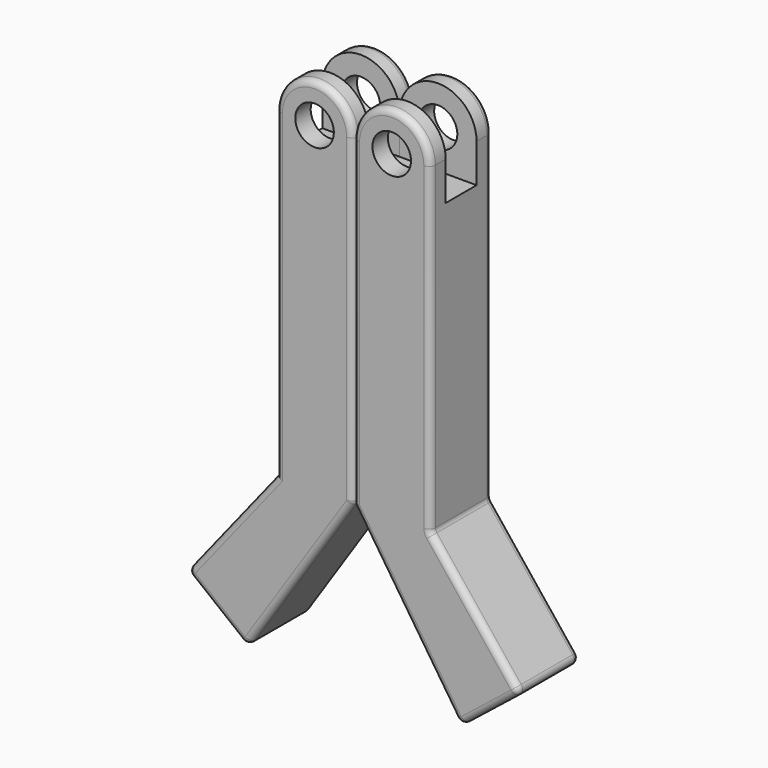
from build123d import *

# Parameters (mm, degrees)
F0_R         = 1.5
F1_DEPTH     = 3
F2_W         = 3
F2_H         = 5.4226633161
F2_H_2       = 3
F3_DEPTH     = 6.001
F5_R         = 0.5
F5_2_R       = 0.5
F6_T1_DEPTH  = 5
F6_T6_DEPTH  = 0.5
F6_T12_DEPTH = 0.5
F7_R         = 0.5


# Not quite as in the source:
# - a fillet or chamfer that OpenCascade refuses, or shapes differently, is made with other operations: its cross-section is extruded or revolved along the edge and cut away or added


with BuildPart() as f1:
    # F0 (on Front) → F1 (new body, symmetric)
    with BuildSketch(Plane.XZ):
        with BuildLine():
            Line((-8.285876948, -12.5037691598), (0, 0))
            Line((0, 0), (0, 25))
            ThreePointArc((0, 25), (-3, 28), (-6, 25))
            Line((-6, 25), (-6, 0))
            Line((-6, 0), (-12.9798034719, -8.766516989))
            Line((-12.9798034719, -8.766516989), (-8.285876948, -12.5037691598))
        make_face()
        with Locations((-3, 25)):
            Circle(F0_R, mode=Mode.SUBTRACT)
    extrude(amount=F1_DEPTH, both=True)

    # F2 (on face) → F3 (cut, through all)
    with BuildSketch(Plane(origin=(-6, 0, 0), x_dir=(0, -1, 0), z_dir=(-1, 0, 0))):
        with Locations((0, 27.7113316581)):
            Rectangle(F2_W, F2_H)
        with Locations((0, 23.5)):
            Rectangle(F2_W, F2_H_2)
    extrude(amount=-F3_DEPTH, mode=Mode.SUBTRACT)


with BuildPart() as f4_1:
    # F4: instance of F1
    add(f1.part.mirror(Plane.YZ))

    # F5
    f5_edges = [f4_1.edges().sort_by_distance(p)[0] for p in [
        (6, -3, 12.5),
        (4.142938, -3, -6.251885),
        (9.489902, -3, -4.383258),
        (9.489902, 3, -4.383258),
        (6, 0, 0),
        (6, 3, 12.5),
        (4.142938, 3, -6.251885),
        (10.63284, 3, -10.635143),
        (12.979803, 0, -8.766517),
        (10.63284, -3, -10.635143),
    ]]
    fillet(f5_edges, radius=F5_R)

    # F6: fillet of radius 0.5 on 1 edges, made by hand

    # F6_s2 → F6_t1 (cut)
    with BuildSketch(Plane.XZ.offset(-2.5)):
        with BuildLine():
            ThreePointArc((7.9844875816, -12.0489587531), (8.3233111968, -12.2666463263), (8.7127175678, -12.1639233985))
            Line((8.7127175678, -12.1639233985), (8.285876948, -12.5037691598))
            Line((8.285876948, -12.5037691598), (7.9844875816, -12.0489587531))
        make_face()
    extrude(amount=F6_T1_DEPTH, mode=Mode.SUBTRACT)


with BuildPart() as f1_1:
    add(f1.part)

    # F5#2
    f5_2_edges = [f1_1.edges().sort_by_distance(p)[0] for p in [
        (-6, -3, 12.5),
        (-4.142938, -3, -6.251885),
        (-9.489902, -3, -4.383258),
        (-10.63284, -3, -10.635143),
        (0, 3, 12.5),
        (-6, 3, 12.5),
        (-9.489902, 3, -4.383258),
        (-4.142938, 3, -6.251885),
        (-10.63284, 3, -10.635143),
        (-8.285877, 0, -12.503769),
        (-12.979803, 0, -8.766517),
    ]]
    fillet(f5_2_edges, radius=F5_2_R)

    # F7
    f7_edges = [f1_1.edges().sort_by_distance(p)[0] for p in [
        (0, 0, 0),
    ]]
    fillet(f7_edges, radius=F7_R)


with BuildPart() as f6_tool4:
    # F6_s5 → F6_t6 (new body)
    with BuildSketch(Plane.XZ.offset(2.5)):
        Polygon((8.4012798869, -11.7727628549), (7.9844875816, -12.0489587531), (8.285876948, -12.5037691598), (8.7127175678, -12.1639233985), align=None)
    extrude(amount=F6_T6_DEPTH)

    # F6_s7 → F6_t8 (revolve, cut)
    with BuildSketch(Plane(origin=(8.4012798869, -2.5, -11.7727628549), x_dir=(0.1559373803, 0, 0.9877669429), z_dir=(0.9877669429, 0, -0.1559373803))):
        with BuildLine():
            ThreePointArc((0, -0.5), (0.5, 0), (0, 0.5))
            Line((0, 0.5), (0, -0.5))
        make_face()
    revolve(axis=Axis((8.4012798869, -2.5, -11.7727628549), (0, -1, 0)), mode=Mode.SUBTRACT)


with BuildPart() as f4_1_1:
    add(f4_1.part)

    # F6_t3: cut F6_tool4
    add(f6_tool4.part, mode=Mode.SUBTRACT)


with BuildPart() as f6_tool10:
    # F6_s11 → F6_t12 (new body)
    with BuildSketch(Plane.XZ.offset(-2.5)):
        Polygon((8.4012798869, -11.7727628549), (7.9844875816, -12.0489587531), (8.285876948, -12.5037691598), (8.7127175678, -12.1639233985), align=None)
    extrude(amount=-F6_T12_DEPTH)

    # F6_s13 → F6_t14 (revolve, cut)
    with BuildSketch(Plane(origin=(8.4012798869, 2.5, -11.7727628549), x_dir=(0.1559373803, 0, 0.9877669429), z_dir=(-0.9877669429, 0, 0.1559373803))):
        with BuildLine():
            ThreePointArc((0, -0.5), (0.5, 0), (0, 0.5))
            Line((0, 0.5), (0, -0.5))
        make_face()
    revolve(axis=Axis((8.4012798869, 2.5, -11.7727628549), (0, 1, 0)), mode=Mode.SUBTRACT)


with BuildPart() as f4_1_2:
    add(f4_1_1.part)

    # F6_t9: cut F6_tool10
    add(f6_tool10.part, mode=Mode.SUBTRACT)


solid = Compound([f1_1.part, f4_1_2.part])
